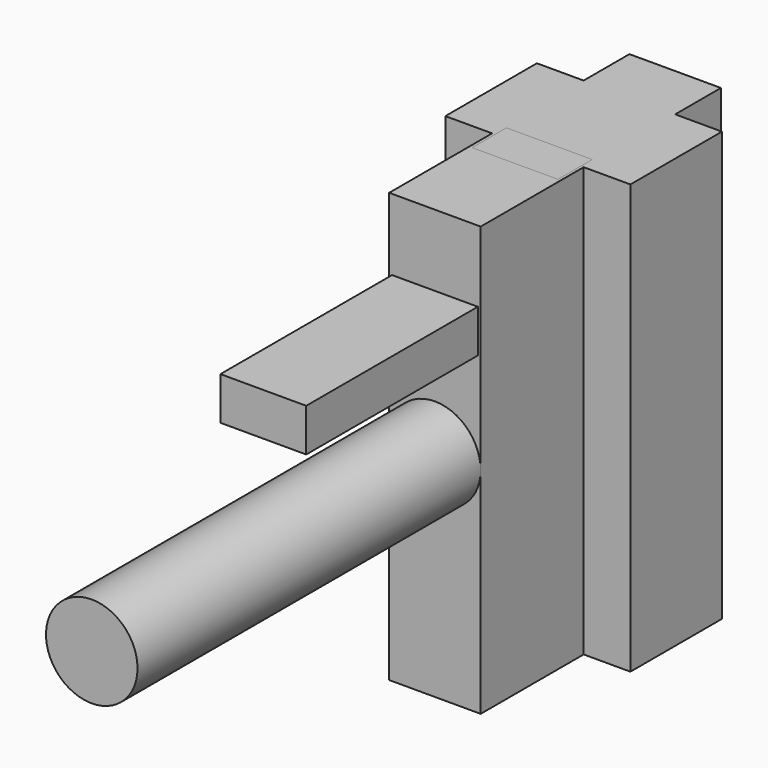
from build123d import *

# Parameters (mm, degrees)
F1_DEPTH = 7.5
F2_R     = 1.6
F3_DEPTH = 15
F4_W     = 3
F4_H     = 1.5
F5_DEPTH = 7.5
F6_W     = 3
F6_H     = 1.5
F7_DEPTH = 7.5


with BuildPart() as f1:
    # F0 (on Top) → F1 (new body, symmetric)
    with BuildSketch(Plane.XY):
        Polygon((1.6, 10.5), (0, 10.5), (-1.6, 10.5), (-1.6, 8.5), (-3.2350461341, 8.5), (-3.2350461341, 4.5), (-1.6, 4.5), (-1.6, 0), (0, 0), (1.6, 0), (1.6, 4.5), (3.2350461341, 4.5), (3.2350461341, 8.5), (1.6, 8.5), align=None)
    extrude(amount=F1_DEPTH, both=True)

    # F2 (on Front) → F3 (join)
    with BuildSketch(Plane.XZ):
        Circle(F2_R)
    extrude(amount=F3_DEPTH)


with BuildPart() as f5:
    # F4 (on Front) → F5 (new body, symmetric)
    with BuildSketch(Plane.XZ):
        with Locations((0, 4.25)):
            Rectangle(F4_W, F4_H)
    extrude(amount=F5_DEPTH, both=True)

    # F6 (on Top) → F7 (join, symmetric)
    with BuildSketch(Plane.XY):
        with Locations((0, 4.25)):
            Rectangle(F6_W, F6_H)
    extrude(amount=F7_DEPTH, both=True)


solid = Compound([f1.part, f5.part])
